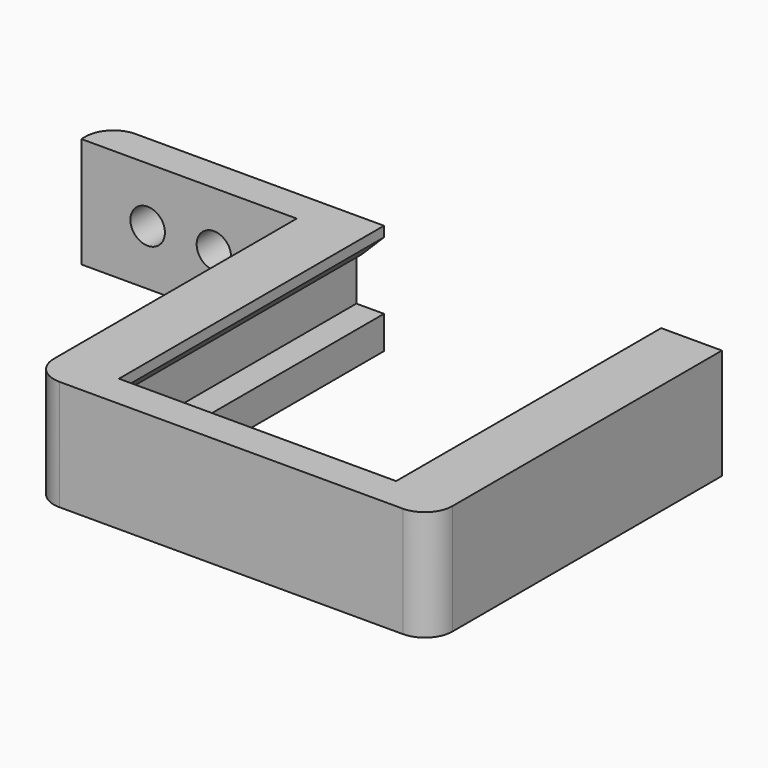
from build123d import *

# Parameters (mm, degrees)
F1_DEPTH    = 20
F3_D        = 6.2484
F4_W        = 60
F4_H        = 6
F6_DEPTH    = 5
F5_W        = 60
F5_H        = 5.8524994925
F5_H_2      = 5.9575000778
F7_DEPTH    = 5
F8_SIZE     = 4
F9_T1_DEPTH = 45
F9_T3_DEPTH = 34.127861456
F9_T5_DEPTH = 34.127861456


# Not quite as in the source:
# - a fillet or chamfer that OpenCascade refuses, or shapes differently, is made with other operations: its cross-section is extruded or revolved along the edge and cut away or added


with BuildPart() as f1:
    # F0 (on Top) → F1 (new body)
    with BuildSketch(Plane.XY):
        Polygon((45, 0), (0, 0), (0, -6), (39, -6), (39, -66), (111.2, -66), (111.2, 0), (105.2, 0), (105.2, -60), (45, -60), align=None)
    extrude(amount=F1_DEPTH)

    # F3 (through all)
    with Locations(Plane(origin=(0, 0, 0), x_dir=(-1, 0, 0), z_dir=(0, 1, 0))):
        with Locations((-36, 10), (-24, 10), (-12, 10)):
            Hole(F3_D / 2)

    # F4 (on face) → F6 (join)
    with BuildSketch(Plane(origin=(105.2, 0, 0), x_dir=(0, -1, 0), z_dir=(-1, 0, 0))):
        with Locations((30, 17)):
            Rectangle(F4_W, F4_H)
        with Locations((30, 3)):
            Rectangle(F4_W, F4_H)
    extrude(amount=F6_DEPTH)

    # F5 (on face) → F7 (join)
    with BuildSketch(Plane.YZ.offset(45)):
        with Locations((-30, 17.0737502538)):
            Rectangle(F5_W, F5_H)
        with Locations((-30, 2.9787500389)):
            Rectangle(F5_W, F5_H_2)
    extrude(amount=F7_DEPTH)

    # F8
    f8_edges = [f1.edges().sort_by_distance(p)[0] for p in [
        (50, -30, 14.147501),
        (100.2, -30, 14),
    ]]
    chamfer(f8_edges, length=F8_SIZE)

    # F9: fillet of radius 5 on 4 edges, made by hand

    # F9_s2 → F9_t1 (cut)
    with BuildSketch(Plane.XY.offset(-12.5)):
        with BuildLine():
            ThreePointArc((106.2, -66), (109.7355339059, -64.5355339059), (111.2, -61))
            Line((111.2, -61), (111.2, -66))
            Line((111.2, -66), (106.2, -66))
        make_face()
        with BuildLine():
            ThreePointArc((5, 0), (1.4644660941, -1.4644660941), (0, -5))
            Line((0, -5), (0, 0))
            Line((0, 0), (5, 0))
        make_face()
    extrude(amount=F9_T1_DEPTH, mode=Mode.SUBTRACT)

    # F9_s4 → F9_t3 (cut)
    with BuildSketch(Plane.XY.offset(-1.627861456)):
        with BuildLine():
            ThreePointArc((39, -61), (40.4644660941, -64.5355339059), (44, -66))
            Line((44, -66), (39, -66))
            Line((39, -66), (39, -61))
        make_face()
    extrude(amount=F9_T3_DEPTH, mode=Mode.SUBTRACT)

    # F9_s6 → F9_t5 (cut)
    with BuildSketch(Plane.XY.offset(-12.5)):
        with BuildLine():
            ThreePointArc((44, -66), (40.4644660941, -64.5355339059), (39, -61))
            Line((39, -61), (39, -66))
            Line((39, -66), (44, -66))
        make_face()
    extrude(amount=F9_T5_DEPTH, mode=Mode.SUBTRACT)


solid = f1.part
